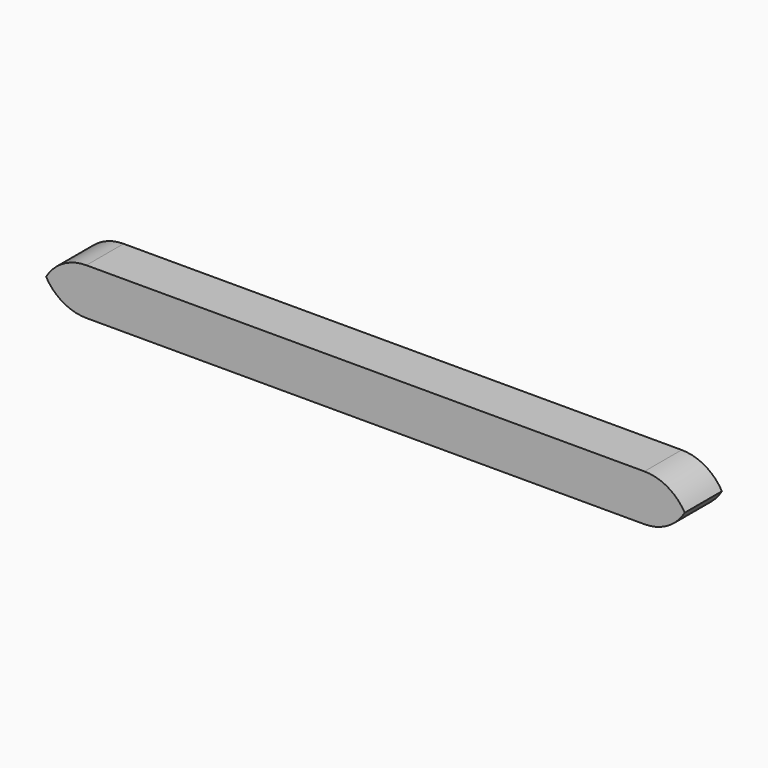
from build123d import *

# Parameters (mm, degrees)
F0_W        = 177.8
F0_H        = 12.7
F1_DEPTH    = 12.7
F2_T1_DEPTH = 76.2


# Not quite as in the source:
# - a fillet or chamfer that OpenCascade refuses, or shapes differently, is made with other operations: its cross-section is extruded or revolved along the edge and cut away or added


with BuildPart() as f1:
    # F0 (on Front) → F1 (new body)
    with BuildSketch(Plane.XZ):
        with Locations((21.4704718173, 53.7259025425)):
            Rectangle(F0_W, F0_H)
    extrude(amount=F1_DEPTH)

    # F2: fillet of radius 12.7 on 4 edges, made by hand

    # F2_s2 → F2_t1 (cut)
    with BuildSketch(Plane.XZ.offset(-31.75)):
        with BuildLine():
            ThreePointArc((-67.4295281827, 47.3759025425), (-63.7097843038, 56.3561586636), (-54.7295281827, 60.0759025425))
            Line((-54.7295281827, 60.0759025425), (-67.4295281827, 60.0759025425))
            Line((-67.4295281827, 60.0759025425), (-67.4295281827, 47.3759025425))
        make_face()
        with BuildLine():
            ThreePointArc((110.3704718173, 47.3759025425), (106.6507279383, 56.3561586636), (97.6704718173, 60.0759025425))
            Line((97.6704718173, 60.0759025425), (110.3704718173, 60.0759025425))
            Line((110.3704718173, 60.0759025425), (110.3704718173, 47.3759025425))
        make_face()
        with BuildLine():
            ThreePointArc((97.6704718173, 47.3759025425), (106.6507279383, 51.0956464214), (110.3704718173, 60.0759025425))
            Line((110.3704718173, 60.0759025425), (110.3704718173, 47.3759025425))
            Line((110.3704718173, 47.3759025425), (97.6704718173, 47.3759025425))
        make_face()
        with BuildLine():
            ThreePointArc((-67.4295281827, 60.0759025425), (-63.7097843038, 51.0956464214), (-54.7295281827, 47.3759025425))
            Line((-54.7295281827, 47.3759025425), (-67.4295281827, 47.3759025425))
            Line((-67.4295281827, 47.3759025425), (-67.4295281827, 60.0759025425))
        make_face()
    extrude(amount=F2_T1_DEPTH, mode=Mode.SUBTRACT)


solid = f1.part
